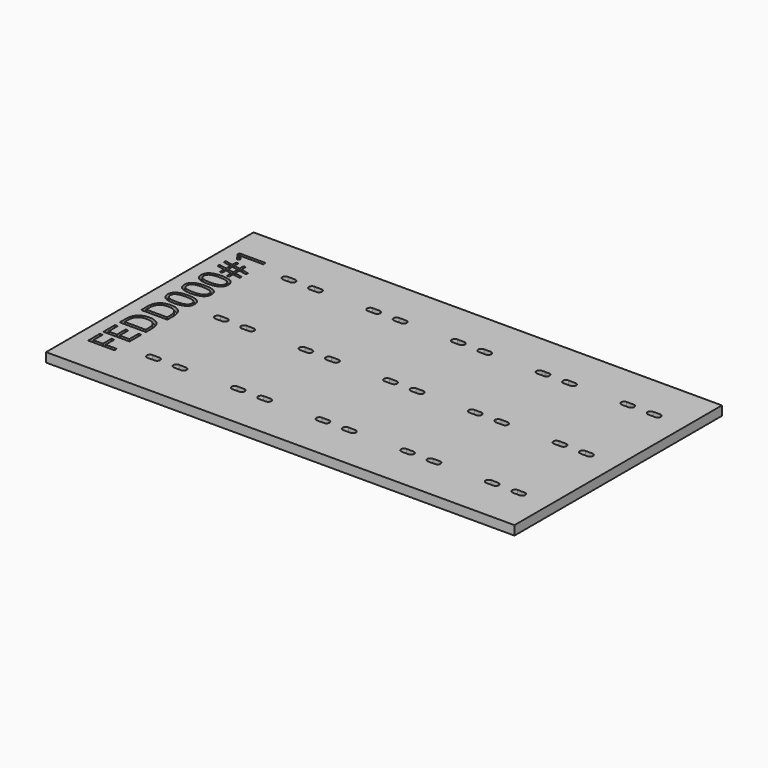
from build123d import *

# Parameters (mm, degrees)
F0_W         = 177
F0_H         = 98
F1_DEPTH     = 3.5
F2_TEXT_SIZE = 13.8888888889
F3_DEPTH     = 1.5
F5_DEPTH     = 3.5
F6_T1_DEPTH  = 3.5


# Not quite as in the source:
# - a fillet or chamfer that OpenCascade refuses, or shapes differently, is made with other operations: its cross-section is extruded or revolved along the edge and cut away or added
# - Text() gives the source's letters only with a copy of the font that has no kerning and outlines rounded to 1/6400 em; it was checked with that copy


with BuildPart() as f1:
    # F0 (on Top) → F1 (new body)
    with BuildSketch(Plane.XY):
        with Locations((0.9526101351, -0.284535466)):
            Rectangle(F0_W, F0_H)
    extrude(amount=F1_DEPTH)

    # F2 (on face) → F3 (cut)
    with BuildSketch(Plane.XY.offset(3.5)):
        with Locations(Location((-72.5473898649, -37.126535466), (0, 0, 90))):
            Text('FEDD000#1', F2_TEXT_SIZE, font='Open Sans', text_align=(TextAlign.LEFT, TextAlign.BOTTOM))
    extrude(amount=-F3_DEPTH, mode=Mode.SUBTRACT)

    # F4 (on face) → F5 (cut, through all)
    with BuildSketch(Plane.XY.offset(3.5)):
        with BuildLine():
            ThreePointArc((-60.5473898649, 30.565464534), (-59.7342170666, 30.9022917356), (-59.3973898649, 31.715464534))
            ThreePointArc((-59.3973898649, 31.715464534), (-59.7342170666, 32.5286373324), (-60.5473898649, 32.865464534))
            ThreePointArc((-60.5473898649, 32.865464534), (-61.6973898649, 31.715464534), (-60.5473898649, 30.565464534))
        make_face()
        with BuildLine():
            ThreePointArc((-60.5473898649, 32.865464534), (-59.7342170666, 32.5286373324), (-59.3973898649, 31.715464534))
            ThreePointArc((-59.3973898649, 31.715464534), (-59.7342170666, 30.9022917356), (-60.5473898649, 30.565464534))
            Line((-60.5473898649, 30.565464534), (-58.0473898649, 30.565464534))
            Line((-58.0473898649, 30.565464534), (-58.0473898649, 32.865464534))
            Line((-58.0473898649, 32.865464534), (-60.5473898649, 32.865464534))
        make_face()
        with BuildLine():
            ThreePointArc((-60.5473898649, 30.565464534), (-61.6973898649, 31.715464534), (-60.5473898649, 32.865464534))
            Line((-60.5473898649, 32.865464534), (-63.0473898649, 32.865464534))
            Line((-63.0473898649, 32.865464534), (-63.0473898649, 30.565464534))
            Line((-63.0473898649, 30.565464534), (-60.5473898649, 30.565464534))
        make_face()
        with BuildLine():
            ThreePointArc((-50.5473898649, 30.565464534), (-49.7342170666, 30.9022917356), (-49.3973898649, 31.715464534))
            ThreePointArc((-49.3973898649, 31.715464534), (-49.7342170666, 32.5286373324), (-50.5473898649, 32.865464534))
            ThreePointArc((-50.5473898649, 32.865464534), (-51.6973898649, 31.715464534), (-50.5473898649, 30.565464534))
        make_face()
        with BuildLine():
            ThreePointArc((-50.5473898649, 32.865464534), (-49.7342170666, 32.5286373324), (-49.3973898649, 31.715464534))
            ThreePointArc((-49.3973898649, 31.715464534), (-49.7342170666, 30.9022917356), (-50.5473898649, 30.565464534))
            Line((-50.5473898649, 30.565464534), (-48.0473898649, 30.565464534))
            Line((-48.0473898649, 30.565464534), (-48.0473898649, 32.865464534))
            Line((-48.0473898649, 32.865464534), (-50.5473898649, 32.865464534))
        make_face()
        with BuildLine():
            ThreePointArc((-50.5473898649, 30.565464534), (-51.6973898649, 31.715464534), (-50.5473898649, 32.865464534))
            Line((-50.5473898649, 32.865464534), (-53.0473898649, 32.865464534))
            Line((-53.0473898649, 32.865464534), (-53.0473898649, 30.565464534))
            Line((-53.0473898649, 30.565464534), (-50.5473898649, 30.565464534))
        make_face()
        with BuildLine():
            ThreePointArc((-28.5473898649, 30.565464534), (-27.7342170666, 30.9022917356), (-27.3973898649, 31.715464534))
            ThreePointArc((-27.3973898649, 31.715464534), (-27.7342170666, 32.5286373324), (-28.5473898649, 32.865464534))
            ThreePointArc((-28.5473898649, 32.865464534), (-29.6973898649, 31.715464534), (-28.5473898649, 30.565464534))
        make_face()
        with BuildLine():
            ThreePointArc((-28.5473898649, 32.865464534), (-27.7342170666, 32.5286373324), (-27.3973898649, 31.715464534))
            ThreePointArc((-27.3973898649, 31.715464534), (-27.7342170666, 30.9022917356), (-28.5473898649, 30.565464534))
            Line((-28.5473898649, 30.565464534), (-26.0473898649, 30.565464534))
            Line((-26.0473898649, 30.565464534), (-26.0473898649, 32.865464534))
            Line((-26.0473898649, 32.865464534), (-28.5473898649, 32.865464534))
        make_face()
        with BuildLine():
            ThreePointArc((-28.5473898649, 30.565464534), (-29.6973898649, 31.715464534), (-28.5473898649, 32.865464534))
            Line((-28.5473898649, 32.865464534), (-31.0473898649, 32.865464534))
            Line((-31.0473898649, 32.865464534), (-31.0473898649, 30.565464534))
            Line((-31.0473898649, 30.565464534), (-28.5473898649, 30.565464534))
        make_face()
        with BuildLine():
            ThreePointArc((-18.5473898649, 30.565464534), (-17.7342170666, 30.9022917356), (-17.3973898649, 31.715464534))
            ThreePointArc((-17.3973898649, 31.715464534), (-17.7342170666, 32.5286373324), (-18.5473898649, 32.865464534))
            ThreePointArc((-18.5473898649, 32.865464534), (-19.6973898649, 31.715464534), (-18.5473898649, 30.565464534))
        make_face()
        with BuildLine():
            ThreePointArc((-18.5473898649, 32.865464534), (-17.7342170666, 32.5286373324), (-17.3973898649, 31.715464534))
            ThreePointArc((-17.3973898649, 31.715464534), (-17.7342170666, 30.9022917356), (-18.5473898649, 30.565464534))
            Line((-18.5473898649, 30.565464534), (-16.0473898649, 30.565464534))
            Line((-16.0473898649, 30.565464534), (-16.0473898649, 32.865464534))
            Line((-16.0473898649, 32.865464534), (-18.5473898649, 32.865464534))
        make_face()
        with BuildLine():
            ThreePointArc((-18.5473898649, 30.565464534), (-19.6973898649, 31.715464534), (-18.5473898649, 32.865464534))
            Line((-18.5473898649, 32.865464534), (-21.0473898649, 32.865464534))
            Line((-21.0473898649, 32.865464534), (-21.0473898649, 30.565464534))
            Line((-21.0473898649, 30.565464534), (-18.5473898649, 30.565464534))
        make_face()
        with BuildLine():
            ThreePointArc((3.4526101351, 30.565464534), (4.2657829334, 30.9022917356), (4.6026101351, 31.715464534))
            ThreePointArc((4.6026101351, 31.715464534), (4.2657829334, 32.5286373324), (3.4526101351, 32.865464534))
            ThreePointArc((3.4526101351, 32.865464534), (2.3026101351, 31.715464534), (3.4526101351, 30.565464534))
        make_face()
        with BuildLine():
            ThreePointArc((3.4526101351, 32.865464534), (4.2657829334, 32.5286373324), (4.6026101351, 31.715464534))
            ThreePointArc((4.6026101351, 31.715464534), (4.2657829334, 30.9022917356), (3.4526101351, 30.565464534))
            Line((3.4526101351, 30.565464534), (5.9526101351, 30.565464534))
            Line((5.9526101351, 30.565464534), (5.9526101351, 32.865464534))
            Line((5.9526101351, 32.865464534), (3.4526101351, 32.865464534))
        make_face()
        with BuildLine():
            ThreePointArc((3.4526101351, 30.565464534), (2.3026101351, 31.715464534), (3.4526101351, 32.865464534))
            Line((3.4526101351, 32.865464534), (0.9526101351, 32.865464534))
            Line((0.9526101351, 32.865464534), (0.9526101351, 30.565464534))
            Line((0.9526101351, 30.565464534), (3.4526101351, 30.565464534))
        make_face()
        with BuildLine():
            ThreePointArc((13.4526101351, 30.565464534), (14.2657829334, 30.9022917356), (14.6026101351, 31.715464534))
            ThreePointArc((14.6026101351, 31.715464534), (14.2657829334, 32.5286373324), (13.4526101351, 32.865464534))
            ThreePointArc((13.4526101351, 32.865464534), (12.3026101351, 31.715464534), (13.4526101351, 30.565464534))
        make_face()
        with BuildLine():
            ThreePointArc((13.4526101351, 32.865464534), (14.2657829334, 32.5286373324), (14.6026101351, 31.715464534))
            ThreePointArc((14.6026101351, 31.715464534), (14.2657829334, 30.9022917356), (13.4526101351, 30.565464534))
            Line((13.4526101351, 30.565464534), (15.9526101351, 30.565464534))
            Line((15.9526101351, 30.565464534), (15.9526101351, 32.865464534))
            Line((15.9526101351, 32.865464534), (13.4526101351, 32.865464534))
        make_face()
        with BuildLine():
            ThreePointArc((13.4526101351, 30.565464534), (12.3026101351, 31.715464534), (13.4526101351, 32.865464534))
            Line((13.4526101351, 32.865464534), (10.9526101351, 32.865464534))
            Line((10.9526101351, 32.865464534), (10.9526101351, 30.565464534))
            Line((10.9526101351, 30.565464534), (13.4526101351, 30.565464534))
        make_face()
        with BuildLine():
            ThreePointArc((35.23906857, 32.845464534), (34.7188093446, 30.8300062346), (36.6026101351, 31.715464534))
            ThreePointArc((36.6026101351, 31.715464534), (36.3380684344, 32.4492653245), (35.6661517001, 32.845464534))
            Line((35.6661517001, 32.845464534), (35.23906857, 32.845464534))
        make_face()
        with BuildLine():
            ThreePointArc((35.6661517001, 32.845464534), (36.3380684344, 32.4492653245), (36.6026101351, 31.715464534))
            ThreePointArc((36.6026101351, 31.715464534), (34.7188093446, 30.8300062346), (35.23906857, 32.845464534))
            Line((35.23906857, 32.845464534), (32.9526101351, 32.845464534))
            Line((32.9526101351, 32.845464534), (32.9526101351, 30.545464534))
            Line((32.9526101351, 30.545464534), (37.9526101351, 30.545464534))
            Line((37.9526101351, 30.545464534), (37.9526101351, 32.845464534))
            Line((37.9526101351, 32.845464534), (35.6661517001, 32.845464534))
        make_face()
        with BuildLine():
            Line((35.23906857, 32.845464534), (35.6661517001, 32.845464534))
            ThreePointArc((35.6661517001, 32.845464534), (35.4526101351, 32.865464534), (35.23906857, 32.845464534))
        make_face()
        with BuildLine():
            ThreePointArc((45.4526101351, 30.565464534), (46.2657829334, 30.9022917356), (46.6026101351, 31.715464534))
            ThreePointArc((46.6026101351, 31.715464534), (46.2657829334, 32.5286373324), (45.4526101351, 32.865464534))
            ThreePointArc((45.4526101351, 32.865464534), (44.3026101351, 31.715464534), (45.4526101351, 30.565464534))
        make_face()
        with BuildLine():
            ThreePointArc((45.4526101351, 32.865464534), (46.2657829334, 32.5286373324), (46.6026101351, 31.715464534))
            ThreePointArc((46.6026101351, 31.715464534), (46.2657829334, 30.9022917356), (45.4526101351, 30.565464534))
            Line((45.4526101351, 30.565464534), (47.9526101351, 30.565464534))
            Line((47.9526101351, 30.565464534), (47.9526101351, 32.865464534))
            Line((47.9526101351, 32.865464534), (45.4526101351, 32.865464534))
        make_face()
        with BuildLine():
            ThreePointArc((45.4526101351, 30.565464534), (44.3026101351, 31.715464534), (45.4526101351, 32.865464534))
            Line((45.4526101351, 32.865464534), (42.9526101351, 32.865464534))
            Line((42.9526101351, 32.865464534), (42.9526101351, 30.565464534))
            Line((42.9526101351, 30.565464534), (45.4526101351, 30.565464534))
        make_face()
        with BuildLine():
            ThreePointArc((67.4526101351, 30.565464534), (68.2657829334, 30.9022917356), (68.6026101351, 31.715464534))
            ThreePointArc((68.6026101351, 31.715464534), (68.2657829334, 32.5286373324), (67.4526101351, 32.865464534))
            ThreePointArc((67.4526101351, 32.865464534), (66.3026101351, 31.715464534), (67.4526101351, 30.565464534))
        make_face()
        with BuildLine():
            ThreePointArc((67.4526101351, 32.865464534), (68.2657829334, 32.5286373324), (68.6026101351, 31.715464534))
            ThreePointArc((68.6026101351, 31.715464534), (68.2657829334, 30.9022917356), (67.4526101351, 30.565464534))
            Line((67.4526101351, 30.565464534), (69.9526101351, 30.565464534))
            Line((69.9526101351, 30.565464534), (69.9526101351, 32.865464534))
            Line((69.9526101351, 32.865464534), (67.4526101351, 32.865464534))
        make_face()
        with BuildLine():
            ThreePointArc((67.4526101351, 30.565464534), (66.3026101351, 31.715464534), (67.4526101351, 32.865464534))
            Line((67.4526101351, 32.865464534), (64.9526101351, 32.865464534))
            Line((64.9526101351, 32.865464534), (64.9526101351, 30.565464534))
            Line((64.9526101351, 30.565464534), (67.4526101351, 30.565464534))
        make_face()
        with BuildLine():
            ThreePointArc((77.4526101351, 30.565464534), (78.2657829334, 30.9022917356), (78.6026101351, 31.715464534))
            ThreePointArc((78.6026101351, 31.715464534), (78.2657829334, 32.5286373324), (77.4526101351, 32.865464534))
            ThreePointArc((77.4526101351, 32.865464534), (76.3026101351, 31.715464534), (77.4526101351, 30.565464534))
        make_face()
        with BuildLine():
            ThreePointArc((77.4526101351, 32.865464534), (78.2657829334, 32.5286373324), (78.6026101351, 31.715464534))
            ThreePointArc((78.6026101351, 31.715464534), (78.2657829334, 30.9022917356), (77.4526101351, 30.565464534))
            Line((77.4526101351, 30.565464534), (79.9526101351, 30.565464534))
            Line((79.9526101351, 30.565464534), (79.9526101351, 32.865464534))
            Line((79.9526101351, 32.865464534), (77.4526101351, 32.865464534))
        make_face()
        with BuildLine():
            ThreePointArc((77.4526101351, 30.565464534), (76.3026101351, 31.715464534), (77.4526101351, 32.865464534))
            Line((77.4526101351, 32.865464534), (74.9526101351, 32.865464534))
            Line((74.9526101351, 32.865464534), (74.9526101351, 30.565464534))
            Line((74.9526101351, 30.565464534), (77.4526101351, 30.565464534))
        make_face()
        with BuildLine():
            ThreePointArc((-60.5473898649, -1.434535466), (-59.7342170666, -1.0977082644), (-59.3973898649, -0.284535466))
            ThreePointArc((-59.3973898649, -0.284535466), (-59.7342170666, 0.5286373324), (-60.5473898649, 0.865464534))
            ThreePointArc((-60.5473898649, 0.865464534), (-61.6973898649, -0.284535466), (-60.5473898649, -1.434535466))
        make_face()
        with BuildLine():
            ThreePointArc((-60.5473898649, 0.865464534), (-59.7342170666, 0.5286373324), (-59.3973898649, -0.284535466))
            ThreePointArc((-59.3973898649, -0.284535466), (-59.7342170666, -1.0977082644), (-60.5473898649, -1.434535466))
            Line((-60.5473898649, -1.434535466), (-58.0473898649, -1.434535466))
            Line((-58.0473898649, -1.434535466), (-58.0473898649, 0.865464534))
            Line((-58.0473898649, 0.865464534), (-60.5473898649, 0.865464534))
        make_face()
        with BuildLine():
            ThreePointArc((-60.5473898649, -1.434535466), (-61.6973898649, -0.284535466), (-60.5473898649, 0.865464534))
            Line((-60.5473898649, 0.865464534), (-63.0473898649, 0.865464534))
            Line((-63.0473898649, 0.865464534), (-63.0473898649, -1.434535466))
            Line((-63.0473898649, -1.434535466), (-60.5473898649, -1.434535466))
        make_face()
        with BuildLine():
            ThreePointArc((-50.5473898649, -1.434535466), (-49.7342170666, -1.0977082644), (-49.3973898649, -0.284535466))
            ThreePointArc((-49.3973898649, -0.284535466), (-49.7342170666, 0.5286373324), (-50.5473898649, 0.865464534))
            ThreePointArc((-50.5473898649, 0.865464534), (-51.6973898649, -0.284535466), (-50.5473898649, -1.434535466))
        make_face()
        with BuildLine():
            ThreePointArc((-50.5473898649, 0.865464534), (-49.7342170666, 0.5286373324), (-49.3973898649, -0.284535466))
            ThreePointArc((-49.3973898649, -0.284535466), (-49.7342170666, -1.0977082644), (-50.5473898649, -1.434535466))
            Line((-50.5473898649, -1.434535466), (-48.0473898649, -1.434535466))
            Line((-48.0473898649, -1.434535466), (-48.0473898649, 0.865464534))
            Line((-48.0473898649, 0.865464534), (-50.5473898649, 0.865464534))
        make_face()
        with BuildLine():
            ThreePointArc((-50.5473898649, -1.434535466), (-51.6973898649, -0.284535466), (-50.5473898649, 0.865464534))
            Line((-50.5473898649, 0.865464534), (-53.0473898649, 0.865464534))
            Line((-53.0473898649, 0.865464534), (-53.0473898649, -1.434535466))
            Line((-53.0473898649, -1.434535466), (-50.5473898649, -1.434535466))
        make_face()
        with BuildLine():
            ThreePointArc((-28.5473898649, -1.434535466), (-27.7342170666, -1.0977082644), (-27.3973898649, -0.284535466))
            ThreePointArc((-27.3973898649, -0.284535466), (-27.7342170666, 0.5286373324), (-28.5473898649, 0.865464534))
            ThreePointArc((-28.5473898649, 0.865464534), (-29.6973898649, -0.284535466), (-28.5473898649, -1.434535466))
        make_face()
        with BuildLine():
            ThreePointArc((-28.5473898649, 0.865464534), (-27.7342170666, 0.5286373324), (-27.3973898649, -0.284535466))
            ThreePointArc((-27.3973898649, -0.284535466), (-27.7342170666, -1.0977082644), (-28.5473898649, -1.434535466))
            Line((-28.5473898649, -1.434535466), (-26.0473898649, -1.434535466))
            Line((-26.0473898649, -1.434535466), (-26.0473898649, 0.865464534))
            Line((-26.0473898649, 0.865464534), (-28.5473898649, 0.865464534))
        make_face()
        with BuildLine():
            ThreePointArc((-28.5473898649, -1.434535466), (-29.6973898649, -0.284535466), (-28.5473898649, 0.865464534))
            Line((-28.5473898649, 0.865464534), (-31.0473898649, 0.865464534))
            Line((-31.0473898649, 0.865464534), (-31.0473898649, -1.434535466))
            Line((-31.0473898649, -1.434535466), (-28.5473898649, -1.434535466))
        make_face()
        with BuildLine():
            ThreePointArc((-18.5473898649, -1.434535466), (-17.7342170666, -1.0977082644), (-17.3973898649, -0.284535466))
            ThreePointArc((-17.3973898649, -0.284535466), (-17.7342170666, 0.5286373324), (-18.5473898649, 0.865464534))
            ThreePointArc((-18.5473898649, 0.865464534), (-19.6973898649, -0.284535466), (-18.5473898649, -1.434535466))
        make_face()
        with BuildLine():
            ThreePointArc((-18.5473898649, 0.865464534), (-17.7342170666, 0.5286373324), (-17.3973898649, -0.284535466))
            ThreePointArc((-17.3973898649, -0.284535466), (-17.7342170666, -1.0977082644), (-18.5473898649, -1.434535466))
            Line((-18.5473898649, -1.434535466), (-16.0473898649, -1.434535466))
            Line((-16.0473898649, -1.434535466), (-16.0473898649, 0.865464534))
            Line((-16.0473898649, 0.865464534), (-18.5473898649, 0.865464534))
        make_face()
        with BuildLine():
            ThreePointArc((-18.5473898649, -1.434535466), (-19.6973898649, -0.284535466), (-18.5473898649, 0.865464534))
            Line((-18.5473898649, 0.865464534), (-21.0473898649, 0.865464534))
            Line((-21.0473898649, 0.865464534), (-21.0473898649, -1.434535466))
            Line((-21.0473898649, -1.434535466), (-18.5473898649, -1.434535466))
        make_face()
        with BuildLine():
            ThreePointArc((3.4526101351, -1.434535466), (4.2657829334, -1.0977082644), (4.6026101351, -0.284535466))
            ThreePointArc((4.6026101351, -0.284535466), (4.2657829334, 0.5286373324), (3.4526101351, 0.865464534))
            ThreePointArc((3.4526101351, 0.865464534), (2.3026101351, -0.284535466), (3.4526101351, -1.434535466))
        make_face()
        with BuildLine():
            ThreePointArc((3.4526101351, 0.865464534), (4.2657829334, 0.5286373324), (4.6026101351, -0.284535466))
            ThreePointArc((4.6026101351, -0.284535466), (4.2657829334, -1.0977082644), (3.4526101351, -1.434535466))
            Line((3.4526101351, -1.434535466), (5.9526101351, -1.434535466))
            Line((5.9526101351, -1.434535466), (5.9526101351, 0.865464534))
            Line((5.9526101351, 0.865464534), (3.4526101351, 0.865464534))
        make_face()
        with BuildLine():
            ThreePointArc((3.4526101351, -1.434535466), (2.3026101351, -0.284535466), (3.4526101351, 0.865464534))
            Line((3.4526101351, 0.865464534), (0.9526101351, 0.865464534))
            Line((0.9526101351, 0.865464534), (0.9526101351, -1.434535466))
            Line((0.9526101351, -1.434535466), (3.4526101351, -1.434535466))
        make_face()
        with BuildLine():
            ThreePointArc((13.4526101351, -1.434535466), (14.2657829334, -1.0977082644), (14.6026101351, -0.284535466))
            ThreePointArc((14.6026101351, -0.284535466), (14.2657829334, 0.5286373324), (13.4526101351, 0.865464534))
            ThreePointArc((13.4526101351, 0.865464534), (12.3026101351, -0.284535466), (13.4526101351, -1.434535466))
        make_face()
        with BuildLine():
            ThreePointArc((13.4526101351, 0.865464534), (14.2657829334, 0.5286373324), (14.6026101351, -0.284535466))
            ThreePointArc((14.6026101351, -0.284535466), (14.2657829334, -1.0977082644), (13.4526101351, -1.434535466))
            Line((13.4526101351, -1.434535466), (15.9526101351, -1.434535466))
            Line((15.9526101351, -1.434535466), (15.9526101351, 0.865464534))
            Line((15.9526101351, 0.865464534), (13.4526101351, 0.865464534))
        make_face()
        with BuildLine():
            ThreePointArc((13.4526101351, -1.434535466), (12.3026101351, -0.284535466), (13.4526101351, 0.865464534))
            Line((13.4526101351, 0.865464534), (10.9526101351, 0.865464534))
            Line((10.9526101351, 0.865464534), (10.9526101351, -1.434535466))
            Line((10.9526101351, -1.434535466), (13.4526101351, -1.434535466))
        make_face()
        with BuildLine():
            ThreePointArc((35.4526101351, -1.434535466), (36.2657829334, -1.0977082644), (36.6026101351, -0.284535466))
            ThreePointArc((36.6026101351, -0.284535466), (36.2657829334, 0.5286373324), (35.4526101351, 0.865464534))
            ThreePointArc((35.4526101351, 0.865464534), (34.3026101351, -0.284535466), (35.4526101351, -1.434535466))
        make_face()
        with BuildLine():
            ThreePointArc((35.4526101351, 0.865464534), (36.2657829334, 0.5286373324), (36.6026101351, -0.284535466))
            ThreePointArc((36.6026101351, -0.284535466), (36.2657829334, -1.0977082644), (35.4526101351, -1.434535466))
            Line((35.4526101351, -1.434535466), (37.9526101351, -1.434535466))
            Line((37.9526101351, -1.434535466), (37.9526101351, 0.865464534))
            Line((37.9526101351, 0.865464534), (35.4526101351, 0.865464534))
        make_face()
        with BuildLine():
            ThreePointArc((35.4526101351, -1.434535466), (34.3026101351, -0.284535466), (35.4526101351, 0.865464534))
            Line((35.4526101351, 0.865464534), (32.9526101351, 0.865464534))
            Line((32.9526101351, 0.865464534), (32.9526101351, -1.434535466))
            Line((32.9526101351, -1.434535466), (35.4526101351, -1.434535466))
        make_face()
        with BuildLine():
            ThreePointArc((45.4526101351, -1.434535466), (46.2657829334, -1.0977082644), (46.6026101351, -0.284535466))
            ThreePointArc((46.6026101351, -0.284535466), (46.2657829334, 0.5286373324), (45.4526101351, 0.865464534))
            ThreePointArc((45.4526101351, 0.865464534), (44.3026101351, -0.284535466), (45.4526101351, -1.434535466))
        make_face()
        with BuildLine():
            ThreePointArc((45.4526101351, 0.865464534), (46.2657829334, 0.5286373324), (46.6026101351, -0.284535466))
            ThreePointArc((46.6026101351, -0.284535466), (46.2657829334, -1.0977082644), (45.4526101351, -1.434535466))
            Line((45.4526101351, -1.434535466), (47.9526101351, -1.434535466))
            Line((47.9526101351, -1.434535466), (47.9526101351, 0.865464534))
            Line((47.9526101351, 0.865464534), (45.4526101351, 0.865464534))
        make_face()
        with BuildLine():
            ThreePointArc((45.4526101351, -1.434535466), (44.3026101351, -0.284535466), (45.4526101351, 0.865464534))
            Line((45.4526101351, 0.865464534), (42.9526101351, 0.865464534))
            Line((42.9526101351, 0.865464534), (42.9526101351, -1.434535466))
            Line((42.9526101351, -1.434535466), (45.4526101351, -1.434535466))
        make_face()
        with BuildLine():
            ThreePointArc((67.4526101351, -1.434535466), (68.2657829334, -1.0977082644), (68.6026101351, -0.284535466))
            ThreePointArc((68.6026101351, -0.284535466), (68.2657829334, 0.5286373324), (67.4526101351, 0.865464534))
            ThreePointArc((67.4526101351, 0.865464534), (66.3026101351, -0.284535466), (67.4526101351, -1.434535466))
        make_face()
        with BuildLine():
            ThreePointArc((67.4526101351, 0.865464534), (68.2657829334, 0.5286373324), (68.6026101351, -0.284535466))
            ThreePointArc((68.6026101351, -0.284535466), (68.2657829334, -1.0977082644), (67.4526101351, -1.434535466))
            Line((67.4526101351, -1.434535466), (69.9526101351, -1.434535466))
            Line((69.9526101351, -1.434535466), (69.9526101351, 0.865464534))
            Line((69.9526101351, 0.865464534), (67.4526101351, 0.865464534))
        make_face()
        with BuildLine():
            ThreePointArc((67.4526101351, -1.434535466), (66.3026101351, -0.284535466), (67.4526101351, 0.865464534))
            Line((67.4526101351, 0.865464534), (64.9526101351, 0.865464534))
            Line((64.9526101351, 0.865464534), (64.9526101351, -1.434535466))
            Line((64.9526101351, -1.434535466), (67.4526101351, -1.434535466))
        make_face()
        with BuildLine():
            ThreePointArc((77.4526101351, -1.434535466), (78.2657829334, -1.0977082644), (78.6026101351, -0.284535466))
            ThreePointArc((78.6026101351, -0.284535466), (78.2657829334, 0.5286373324), (77.4526101351, 0.865464534))
            ThreePointArc((77.4526101351, 0.865464534), (76.3026101351, -0.284535466), (77.4526101351, -1.434535466))
        make_face()
        with BuildLine():
            ThreePointArc((77.4526101351, 0.865464534), (78.2657829334, 0.5286373324), (78.6026101351, -0.284535466))
            ThreePointArc((78.6026101351, -0.284535466), (78.2657829334, -1.0977082644), (77.4526101351, -1.434535466))
            Line((77.4526101351, -1.434535466), (79.9526101351, -1.434535466))
            Line((79.9526101351, -1.434535466), (79.9526101351, 0.865464534))
            Line((79.9526101351, 0.865464534), (77.4526101351, 0.865464534))
        make_face()
        with BuildLine():
            ThreePointArc((77.4526101351, -1.434535466), (76.3026101351, -0.284535466), (77.4526101351, 0.865464534))
            Line((77.4526101351, 0.865464534), (74.9526101351, 0.865464534))
            Line((74.9526101351, 0.865464534), (74.9526101351, -1.434535466))
            Line((74.9526101351, -1.434535466), (77.4526101351, -1.434535466))
        make_face()
        with BuildLine():
            ThreePointArc((-60.5473898649, -33.434535466), (-59.7342170666, -33.0977082644), (-59.3973898649, -32.284535466))
            ThreePointArc((-59.3973898649, -32.284535466), (-59.7342170666, -31.4713626676), (-60.5473898649, -31.134535466))
            ThreePointArc((-60.5473898649, -31.134535466), (-61.6973898649, -32.284535466), (-60.5473898649, -33.434535466))
        make_face()
        with BuildLine():
            ThreePointArc((-60.5473898649, -31.134535466), (-59.7342170666, -31.4713626676), (-59.3973898649, -32.284535466))
            ThreePointArc((-59.3973898649, -32.284535466), (-59.7342170666, -33.0977082644), (-60.5473898649, -33.434535466))
            Line((-60.5473898649, -33.434535466), (-58.0473898649, -33.434535466))
            Line((-58.0473898649, -33.434535466), (-58.0473898649, -31.134535466))
            Line((-58.0473898649, -31.134535466), (-60.5473898649, -31.134535466))
        make_face()
        with BuildLine():
            ThreePointArc((-60.5473898649, -33.434535466), (-61.6973898649, -32.284535466), (-60.5473898649, -31.134535466))
            Line((-60.5473898649, -31.134535466), (-63.0473898649, -31.134535466))
            Line((-63.0473898649, -31.134535466), (-63.0473898649, -33.434535466))
            Line((-63.0473898649, -33.434535466), (-60.5473898649, -33.434535466))
        make_face()
        with BuildLine():
            ThreePointArc((-50.5473898649, -33.434535466), (-49.7342170666, -33.0977082644), (-49.3973898649, -32.284535466))
            ThreePointArc((-49.3973898649, -32.284535466), (-49.7342170666, -31.4713626676), (-50.5473898649, -31.134535466))
            ThreePointArc((-50.5473898649, -31.134535466), (-51.6973898649, -32.284535466), (-50.5473898649, -33.434535466))
        make_face()
        with BuildLine():
            ThreePointArc((-50.5473898649, -31.134535466), (-49.7342170666, -31.4713626676), (-49.3973898649, -32.284535466))
            ThreePointArc((-49.3973898649, -32.284535466), (-49.7342170666, -33.0977082644), (-50.5473898649, -33.434535466))
            Line((-50.5473898649, -33.434535466), (-48.0473898649, -33.434535466))
            Line((-48.0473898649, -33.434535466), (-48.0473898649, -31.134535466))
            Line((-48.0473898649, -31.134535466), (-50.5473898649, -31.134535466))
        make_face()
        with BuildLine():
            ThreePointArc((-50.5473898649, -33.434535466), (-51.6973898649, -32.284535466), (-50.5473898649, -31.134535466))
            Line((-50.5473898649, -31.134535466), (-53.0473898649, -31.134535466))
            Line((-53.0473898649, -31.134535466), (-53.0473898649, -33.434535466))
            Line((-53.0473898649, -33.434535466), (-50.5473898649, -33.434535466))
        make_face()
        with BuildLine():
            ThreePointArc((-28.5473898649, -33.434535466), (-27.7342170666, -33.0977082644), (-27.3973898649, -32.284535466))
            ThreePointArc((-27.3973898649, -32.284535466), (-27.7342170666, -31.4713626676), (-28.5473898649, -31.134535466))
            ThreePointArc((-28.5473898649, -31.134535466), (-29.6973898649, -32.284535466), (-28.5473898649, -33.434535466))
        make_face()
        with BuildLine():
            ThreePointArc((-28.5473898649, -31.134535466), (-27.7342170666, -31.4713626676), (-27.3973898649, -32.284535466))
            ThreePointArc((-27.3973898649, -32.284535466), (-27.7342170666, -33.0977082644), (-28.5473898649, -33.434535466))
            Line((-28.5473898649, -33.434535466), (-26.0473898649, -33.434535466))
            Line((-26.0473898649, -33.434535466), (-26.0473898649, -31.134535466))
            Line((-26.0473898649, -31.134535466), (-28.5473898649, -31.134535466))
        make_face()
        with BuildLine():
            ThreePointArc((-28.5473898649, -33.434535466), (-29.6973898649, -32.284535466), (-28.5473898649, -31.134535466))
            Line((-28.5473898649, -31.134535466), (-31.0473898649, -31.134535466))
            Line((-31.0473898649, -31.134535466), (-31.0473898649, -33.434535466))
            Line((-31.0473898649, -33.434535466), (-28.5473898649, -33.434535466))
        make_face()
        with BuildLine():
            ThreePointArc((-18.5473898649, -33.434535466), (-17.7342170666, -33.0977082644), (-17.3973898649, -32.284535466))
            ThreePointArc((-17.3973898649, -32.284535466), (-17.7342170666, -31.4713626676), (-18.5473898649, -31.134535466))
            ThreePointArc((-18.5473898649, -31.134535466), (-19.6973898649, -32.284535466), (-18.5473898649, -33.434535466))
        make_face()
        with BuildLine():
            ThreePointArc((-18.5473898649, -31.134535466), (-17.7342170666, -31.4713626676), (-17.3973898649, -32.284535466))
            ThreePointArc((-17.3973898649, -32.284535466), (-17.7342170666, -33.0977082644), (-18.5473898649, -33.434535466))
            Line((-18.5473898649, -33.434535466), (-16.0473898649, -33.434535466))
            Line((-16.0473898649, -33.434535466), (-16.0473898649, -31.134535466))
            Line((-16.0473898649, -31.134535466), (-18.5473898649, -31.134535466))
        make_face()
        with BuildLine():
            ThreePointArc((-18.5473898649, -33.434535466), (-19.6973898649, -32.284535466), (-18.5473898649, -31.134535466))
            Line((-18.5473898649, -31.134535466), (-21.0473898649, -31.134535466))
            Line((-21.0473898649, -31.134535466), (-21.0473898649, -33.434535466))
            Line((-21.0473898649, -33.434535466), (-18.5473898649, -33.434535466))
        make_face()
        with BuildLine():
            ThreePointArc((3.4526101351, -33.434535466), (4.2657829334, -33.0977082644), (4.6026101351, -32.284535466))
            ThreePointArc((4.6026101351, -32.284535466), (4.2657829334, -31.4713626676), (3.4526101351, -31.134535466))
            ThreePointArc((3.4526101351, -31.134535466), (2.3026101351, -32.284535466), (3.4526101351, -33.434535466))
        make_face()
        with BuildLine():
            ThreePointArc((3.4526101351, -31.134535466), (4.2657829334, -31.4713626676), (4.6026101351, -32.284535466))
            ThreePointArc((4.6026101351, -32.284535466), (4.2657829334, -33.0977082644), (3.4526101351, -33.434535466))
            Line((3.4526101351, -33.434535466), (5.9526101351, -33.434535466))
            Line((5.9526101351, -33.434535466), (5.9526101351, -31.134535466))
            Line((5.9526101351, -31.134535466), (3.4526101351, -31.134535466))
        make_face()
        with BuildLine():
            ThreePointArc((3.4526101351, -33.434535466), (2.3026101351, -32.284535466), (3.4526101351, -31.134535466))
            Line((3.4526101351, -31.134535466), (0.9526101351, -31.134535466))
            Line((0.9526101351, -31.134535466), (0.9526101351, -33.434535466))
            Line((0.9526101351, -33.434535466), (3.4526101351, -33.434535466))
        make_face()
        with BuildLine():
            ThreePointArc((13.4526101351, -33.434535466), (14.2657829334, -33.0977082644), (14.6026101351, -32.284535466))
            ThreePointArc((14.6026101351, -32.284535466), (14.2657829334, -31.4713626676), (13.4526101351, -31.134535466))
            ThreePointArc((13.4526101351, -31.134535466), (12.3026101351, -32.284535466), (13.4526101351, -33.434535466))
        make_face()
        with BuildLine():
            ThreePointArc((13.4526101351, -31.134535466), (14.2657829334, -31.4713626676), (14.6026101351, -32.284535466))
            ThreePointArc((14.6026101351, -32.284535466), (14.2657829334, -33.0977082644), (13.4526101351, -33.434535466))
            Line((13.4526101351, -33.434535466), (15.9526101351, -33.434535466))
            Line((15.9526101351, -33.434535466), (15.9526101351, -31.134535466))
            Line((15.9526101351, -31.134535466), (13.4526101351, -31.134535466))
        make_face()
        with BuildLine():
            ThreePointArc((13.4526101351, -33.434535466), (12.3026101351, -32.284535466), (13.4526101351, -31.134535466))
            Line((13.4526101351, -31.134535466), (10.9526101351, -31.134535466))
            Line((10.9526101351, -31.134535466), (10.9526101351, -33.434535466))
            Line((10.9526101351, -33.434535466), (13.4526101351, -33.434535466))
        make_face()
        with BuildLine():
            ThreePointArc((35.4526101351, -33.434535466), (36.2657829334, -33.0977082644), (36.6026101351, -32.284535466))
            ThreePointArc((36.6026101351, -32.284535466), (36.2657829334, -31.4713626676), (35.4526101351, -31.134535466))
            ThreePointArc((35.4526101351, -31.134535466), (34.3026101351, -32.284535466), (35.4526101351, -33.434535466))
        make_face()
        with BuildLine():
            ThreePointArc((35.4526101351, -31.134535466), (36.2657829334, -31.4713626676), (36.6026101351, -32.284535466))
            ThreePointArc((36.6026101351, -32.284535466), (36.2657829334, -33.0977082644), (35.4526101351, -33.434535466))
            Line((35.4526101351, -33.434535466), (37.9526101351, -33.434535466))
            Line((37.9526101351, -33.434535466), (37.9526101351, -31.134535466))
            Line((37.9526101351, -31.134535466), (35.4526101351, -31.134535466))
        make_face()
        with BuildLine():
            ThreePointArc((35.4526101351, -33.434535466), (34.3026101351, -32.284535466), (35.4526101351, -31.134535466))
            Line((35.4526101351, -31.134535466), (32.9526101351, -31.134535466))
            Line((32.9526101351, -31.134535466), (32.9526101351, -33.434535466))
            Line((32.9526101351, -33.434535466), (35.4526101351, -33.434535466))
        make_face()
        with BuildLine():
            ThreePointArc((45.4526101351, -33.434535466), (46.2657829334, -33.0977082644), (46.6026101351, -32.284535466))
            ThreePointArc((46.6026101351, -32.284535466), (46.2657829334, -31.4713626676), (45.4526101351, -31.134535466))
            ThreePointArc((45.4526101351, -31.134535466), (44.3026101351, -32.284535466), (45.4526101351, -33.434535466))
        make_face()
        with BuildLine():
            ThreePointArc((45.4526101351, -31.134535466), (46.2657829334, -31.4713626676), (46.6026101351, -32.284535466))
            ThreePointArc((46.6026101351, -32.284535466), (46.2657829334, -33.0977082644), (45.4526101351, -33.434535466))
            Line((45.4526101351, -33.434535466), (47.9526101351, -33.434535466))
            Line((47.9526101351, -33.434535466), (47.9526101351, -31.134535466))
            Line((47.9526101351, -31.134535466), (45.4526101351, -31.134535466))
        make_face()
        with BuildLine():
            ThreePointArc((45.4526101351, -33.434535466), (44.3026101351, -32.284535466), (45.4526101351, -31.134535466))
            Line((45.4526101351, -31.134535466), (42.9526101351, -31.134535466))
            Line((42.9526101351, -31.134535466), (42.9526101351, -33.434535466))
            Line((42.9526101351, -33.434535466), (45.4526101351, -33.434535466))
        make_face()
        with BuildLine():
            ThreePointArc((67.4526101351, -33.434535466), (68.2657829334, -33.0977082644), (68.6026101351, -32.284535466))
            ThreePointArc((68.6026101351, -32.284535466), (68.2657829334, -31.4713626676), (67.4526101351, -31.134535466))
            ThreePointArc((67.4526101351, -31.134535466), (66.3026101351, -32.284535466), (67.4526101351, -33.434535466))
        make_face()
        with BuildLine():
            ThreePointArc((67.4526101351, -31.134535466), (68.2657829334, -31.4713626676), (68.6026101351, -32.284535466))
            ThreePointArc((68.6026101351, -32.284535466), (68.2657829334, -33.0977082644), (67.4526101351, -33.434535466))
            Line((67.4526101351, -33.434535466), (69.9526101351, -33.434535466))
            Line((69.9526101351, -33.434535466), (69.9526101351, -31.134535466))
            Line((69.9526101351, -31.134535466), (67.4526101351, -31.134535466))
        make_face()
        with BuildLine():
            ThreePointArc((67.4526101351, -33.434535466), (66.3026101351, -32.284535466), (67.4526101351, -31.134535466))
            Line((67.4526101351, -31.134535466), (64.9526101351, -31.134535466))
            Line((64.9526101351, -31.134535466), (64.9526101351, -33.434535466))
            Line((64.9526101351, -33.434535466), (67.4526101351, -33.434535466))
        make_face()
        with BuildLine():
            ThreePointArc((77.4526101351, -33.434535466), (78.2657829334, -33.0977082644), (78.6026101351, -32.284535466))
            ThreePointArc((78.6026101351, -32.284535466), (78.2657829334, -31.4713626676), (77.4526101351, -31.134535466))
            ThreePointArc((77.4526101351, -31.134535466), (76.3026101351, -32.284535466), (77.4526101351, -33.434535466))
        make_face()
        with BuildLine():
            ThreePointArc((77.4526101351, -31.134535466), (78.2657829334, -31.4713626676), (78.6026101351, -32.284535466))
            ThreePointArc((78.6026101351, -32.284535466), (78.2657829334, -33.0977082644), (77.4526101351, -33.434535466))
            Line((77.4526101351, -33.434535466), (79.9526101351, -33.434535466))
            Line((79.9526101351, -33.434535466), (79.9526101351, -31.134535466))
            Line((79.9526101351, -31.134535466), (77.4526101351, -31.134535466))
        make_face()
        with BuildLine():
            ThreePointArc((77.4526101351, -33.434535466), (76.3026101351, -32.284535466), (77.4526101351, -31.134535466))
            Line((77.4526101351, -31.134535466), (74.9526101351, -31.134535466))
            Line((74.9526101351, -31.134535466), (74.9526101351, -33.434535466))
            Line((74.9526101351, -33.434535466), (77.4526101351, -33.434535466))
        make_face()
    extrude(amount=-F5_DEPTH, mode=Mode.SUBTRACT)

    # F6: fillet of radius 1.2 on 120 edges, made by hand

    # F6_s2 → F6_t1 (join)
    with BuildSketch(Plane.XY):
        with BuildLine():
            ThreePointArc((-51.8473898649, 32.865464534), (-52.6959180023, 32.5139926714), (-53.0473898649, 31.665464534))
            Line((-53.0473898649, 31.665464534), (-53.0473898649, 32.865464534))
            Line((-53.0473898649, 32.865464534), (-51.8473898649, 32.865464534))
        make_face()
        with BuildLine():
            ThreePointArc((-48.0473898649, 31.665464534), (-48.3988617275, 32.5139926714), (-49.2473898649, 32.865464534))
            Line((-49.2473898649, 32.865464534), (-48.0473898649, 32.865464534))
            Line((-48.0473898649, 32.865464534), (-48.0473898649, 31.665464534))
        make_face()
        with BuildLine():
            ThreePointArc((-48.0473898649, 31.765464534), (-48.3988617275, 30.9169363966), (-49.2473898649, 30.565464534))
            Line((-49.2473898649, 30.565464534), (-48.0473898649, 30.565464534))
            Line((-48.0473898649, 30.565464534), (-48.0473898649, 31.765464534))
        make_face()
        with BuildLine():
            ThreePointArc((-53.0473898649, 31.765464534), (-52.6959180023, 30.9169363966), (-51.8473898649, 30.565464534))
            Line((-51.8473898649, 30.565464534), (-53.0473898649, 30.565464534))
            Line((-53.0473898649, 30.565464534), (-53.0473898649, 31.765464534))
        make_face()
        with BuildLine():
            ThreePointArc((-61.8473898649, 32.865464534), (-62.6959180023, 32.5139926714), (-63.0473898649, 31.665464534))
            Line((-63.0473898649, 31.665464534), (-63.0473898649, 32.865464534))
            Line((-63.0473898649, 32.865464534), (-61.8473898649, 32.865464534))
        make_face()
        with BuildLine():
            ThreePointArc((-61.8473898649, 0.865464534), (-62.6959180023, 0.5139926714), (-63.0473898649, -0.334535466))
            Line((-63.0473898649, -0.334535466), (-63.0473898649, 0.865464534))
            Line((-63.0473898649, 0.865464534), (-61.8473898649, 0.865464534))
        make_face()
        with BuildLine():
            ThreePointArc((-51.8473898649, 0.865464534), (-52.6959180023, 0.5139926714), (-53.0473898649, -0.334535466))
            Line((-53.0473898649, -0.334535466), (-53.0473898649, 0.865464534))
            Line((-53.0473898649, 0.865464534), (-51.8473898649, 0.865464534))
        make_face()
        with BuildLine():
            ThreePointArc((-29.8473898649, 0.865464534), (-30.6959180023, 0.5139926714), (-31.0473898649, -0.334535466))
            Line((-31.0473898649, -0.334535466), (-31.0473898649, 0.865464534))
            Line((-31.0473898649, 0.865464534), (-29.8473898649, 0.865464534))
        make_face()
        with BuildLine():
            ThreePointArc((-19.8473898649, 0.865464534), (-20.6959180023, 0.5139926714), (-21.0473898649, -0.334535466))
            Line((-21.0473898649, -0.334535466), (-21.0473898649, 0.865464534))
            Line((-21.0473898649, 0.865464534), (-19.8473898649, 0.865464534))
        make_face()
        with BuildLine():
            ThreePointArc((-29.8473898649, 32.865464534), (-30.6959180023, 32.5139926714), (-31.0473898649, 31.665464534))
            Line((-31.0473898649, 31.665464534), (-31.0473898649, 32.865464534))
            Line((-31.0473898649, 32.865464534), (-29.8473898649, 32.865464534))
        make_face()
        with BuildLine():
            ThreePointArc((-19.8473898649, 32.865464534), (-20.6959180023, 32.5139926714), (-21.0473898649, 31.665464534))
            Line((-21.0473898649, 31.665464534), (-21.0473898649, 32.865464534))
            Line((-21.0473898649, 32.865464534), (-19.8473898649, 32.865464534))
        make_face()
        with BuildLine():
            ThreePointArc((-61.8473898649, -31.134535466), (-62.6959180023, -31.4860073286), (-63.0473898649, -32.334535466))
            Line((-63.0473898649, -32.334535466), (-63.0473898649, -31.134535466))
            Line((-63.0473898649, -31.134535466), (-61.8473898649, -31.134535466))
        make_face()
        with BuildLine():
            ThreePointArc((-51.8473898649, -31.134535466), (-52.6959180023, -31.4860073286), (-53.0473898649, -32.334535466))
            Line((-53.0473898649, -32.334535466), (-53.0473898649, -31.134535466))
            Line((-53.0473898649, -31.134535466), (-51.8473898649, -31.134535466))
        make_face()
        with BuildLine():
            ThreePointArc((-29.8473898649, -31.134535466), (-30.6959180023, -31.4860073286), (-31.0473898649, -32.334535466))
            Line((-31.0473898649, -32.334535466), (-31.0473898649, -31.134535466))
            Line((-31.0473898649, -31.134535466), (-29.8473898649, -31.134535466))
        make_face()
        with BuildLine():
            ThreePointArc((-19.8473898649, -31.134535466), (-20.6959180023, -31.4860073286), (-21.0473898649, -32.334535466))
            Line((-21.0473898649, -32.334535466), (-21.0473898649, -31.134535466))
            Line((-21.0473898649, -31.134535466), (-19.8473898649, -31.134535466))
        make_face()
        with BuildLine():
            ThreePointArc((2.1526101351, -31.134535466), (1.3040819977, -31.4860073286), (0.9526101351, -32.334535466))
            Line((0.9526101351, -32.334535466), (0.9526101351, -31.134535466))
            Line((0.9526101351, -31.134535466), (2.1526101351, -31.134535466))
        make_face()
        with BuildLine():
            ThreePointArc((12.1526101351, -31.134535466), (11.3040819977, -31.4860073286), (10.9526101351, -32.334535466))
            Line((10.9526101351, -32.334535466), (10.9526101351, -31.134535466))
            Line((10.9526101351, -31.134535466), (12.1526101351, -31.134535466))
        make_face()
        with BuildLine():
            ThreePointArc((2.1526101351, 32.865464534), (1.3040819977, 32.5139926714), (0.9526101351, 31.665464534))
            Line((0.9526101351, 31.665464534), (0.9526101351, 32.865464534))
            Line((0.9526101351, 32.865464534), (2.1526101351, 32.865464534))
        make_face()
        with BuildLine():
            ThreePointArc((12.1526101351, 32.865464534), (11.3040819977, 32.5139926714), (10.9526101351, 31.665464534))
            Line((10.9526101351, 31.665464534), (10.9526101351, 32.865464534))
            Line((10.9526101351, 32.865464534), (12.1526101351, 32.865464534))
        make_face()
        with BuildLine():
            ThreePointArc((34.1526101351, 32.845464534), (33.3040819977, 32.4939926714), (32.9526101351, 31.645464534))
            Line((32.9526101351, 31.645464534), (32.9526101351, 32.845464534))
            Line((32.9526101351, 32.845464534), (34.1526101351, 32.845464534))
        make_face()
        with BuildLine():
            ThreePointArc((44.1526101351, 32.865464534), (43.3040819977, 32.5139926714), (42.9526101351, 31.665464534))
            Line((42.9526101351, 31.665464534), (42.9526101351, 32.865464534))
            Line((42.9526101351, 32.865464534), (44.1526101351, 32.865464534))
        make_face()
        with BuildLine():
            ThreePointArc((66.1526101351, 32.865464534), (65.3040819977, 32.5139926714), (64.9526101351, 31.665464534))
            Line((64.9526101351, 31.665464534), (64.9526101351, 32.865464534))
            Line((64.9526101351, 32.865464534), (66.1526101351, 32.865464534))
        make_face()
        with BuildLine():
            ThreePointArc((76.1526101351, 32.865464534), (75.3040819977, 32.5139926714), (74.9526101351, 31.665464534))
            Line((74.9526101351, 31.665464534), (74.9526101351, 32.865464534))
            Line((74.9526101351, 32.865464534), (76.1526101351, 32.865464534))
        make_face()
        with BuildLine():
            ThreePointArc((66.1526101351, -31.134535466), (65.3040819977, -31.4860073286), (64.9526101351, -32.334535466))
            Line((64.9526101351, -32.334535466), (64.9526101351, -31.134535466))
            Line((64.9526101351, -31.134535466), (66.1526101351, -31.134535466))
        make_face()
        with BuildLine():
            ThreePointArc((44.1526101351, -31.134535466), (43.3040819977, -31.4860073286), (42.9526101351, -32.334535466))
            Line((42.9526101351, -32.334535466), (42.9526101351, -31.134535466))
            Line((42.9526101351, -31.134535466), (44.1526101351, -31.134535466))
        make_face()
        with BuildLine():
            ThreePointArc((34.1526101351, -31.134535466), (33.3040819977, -31.4860073286), (32.9526101351, -32.334535466))
            Line((32.9526101351, -32.334535466), (32.9526101351, -31.134535466))
            Line((32.9526101351, -31.134535466), (34.1526101351, -31.134535466))
        make_face()
        with BuildLine():
            ThreePointArc((2.1526101351, 0.865464534), (1.3040819977, 0.5139926714), (0.9526101351, -0.334535466))
            Line((0.9526101351, -0.334535466), (0.9526101351, 0.865464534))
            Line((0.9526101351, 0.865464534), (2.1526101351, 0.865464534))
        make_face()
        with BuildLine():
            ThreePointArc((12.1526101351, 0.865464534), (11.3040819977, 0.5139926714), (10.9526101351, -0.334535466))
            Line((10.9526101351, -0.334535466), (10.9526101351, 0.865464534))
            Line((10.9526101351, 0.865464534), (12.1526101351, 0.865464534))
        make_face()
        with BuildLine():
            ThreePointArc((34.1526101351, 0.865464534), (33.3040819977, 0.5139926714), (32.9526101351, -0.334535466))
            Line((32.9526101351, -0.334535466), (32.9526101351, 0.865464534))
            Line((32.9526101351, 0.865464534), (34.1526101351, 0.865464534))
        make_face()
        with BuildLine():
            ThreePointArc((44.1526101351, 0.865464534), (43.3040819977, 0.5139926714), (42.9526101351, -0.334535466))
            Line((42.9526101351, -0.334535466), (42.9526101351, 0.865464534))
            Line((42.9526101351, 0.865464534), (44.1526101351, 0.865464534))
        make_face()
        with BuildLine():
            ThreePointArc((66.1526101351, 0.865464534), (65.3040819977, 0.5139926714), (64.9526101351, -0.334535466))
            Line((64.9526101351, -0.334535466), (64.9526101351, 0.865464534))
            Line((64.9526101351, 0.865464534), (66.1526101351, 0.865464534))
        make_face()
        with BuildLine():
            ThreePointArc((76.1526101351, 0.865464534), (75.3040819977, 0.5139926714), (74.9526101351, -0.334535466))
            Line((74.9526101351, -0.334535466), (74.9526101351, 0.865464534))
            Line((74.9526101351, 0.865464534), (76.1526101351, 0.865464534))
        make_face()
        with BuildLine():
            ThreePointArc((76.1526101351, -31.134535466), (75.3040819977, -31.4860073286), (74.9526101351, -32.334535466))
            Line((74.9526101351, -32.334535466), (74.9526101351, -31.134535466))
            Line((74.9526101351, -31.134535466), (76.1526101351, -31.134535466))
        make_face()
        with BuildLine():
            ThreePointArc((-58.0473898649, 31.665464534), (-58.3988617275, 32.5139926714), (-59.2473898649, 32.865464534))
            Line((-59.2473898649, 32.865464534), (-58.0473898649, 32.865464534))
            Line((-58.0473898649, 32.865464534), (-58.0473898649, 31.665464534))
        make_face()
        with BuildLine():
            ThreePointArc((-26.0473898649, 31.665464534), (-26.3988617275, 32.5139926714), (-27.2473898649, 32.865464534))
            Line((-27.2473898649, 32.865464534), (-26.0473898649, 32.865464534))
            Line((-26.0473898649, 32.865464534), (-26.0473898649, 31.665464534))
        make_face()
        with BuildLine():
            ThreePointArc((-16.0473898649, 31.665464534), (-16.3988617275, 32.5139926714), (-17.2473898649, 32.865464534))
            Line((-17.2473898649, 32.865464534), (-16.0473898649, 32.865464534))
            Line((-16.0473898649, 32.865464534), (-16.0473898649, 31.665464534))
        make_face()
        with BuildLine():
            ThreePointArc((-16.0473898649, -0.334535466), (-16.3988617275, 0.5139926714), (-17.2473898649, 0.865464534))
            Line((-17.2473898649, 0.865464534), (-16.0473898649, 0.865464534))
            Line((-16.0473898649, 0.865464534), (-16.0473898649, -0.334535466))
        make_face()
        with BuildLine():
            ThreePointArc((-48.0473898649, -0.334535466), (-48.3988617275, 0.5139926714), (-49.2473898649, 0.865464534))
            Line((-49.2473898649, 0.865464534), (-48.0473898649, 0.865464534))
            Line((-48.0473898649, 0.865464534), (-48.0473898649, -0.334535466))
        make_face()
        with BuildLine():
            ThreePointArc((-58.0473898649, -0.334535466), (-58.3988617275, 0.5139926714), (-59.2473898649, 0.865464534))
            Line((-59.2473898649, 0.865464534), (-58.0473898649, 0.865464534))
            Line((-58.0473898649, 0.865464534), (-58.0473898649, -0.334535466))
        make_face()
        with BuildLine():
            ThreePointArc((-58.0473898649, -32.334535466), (-58.3988617275, -31.4860073286), (-59.2473898649, -31.134535466))
            Line((-59.2473898649, -31.134535466), (-58.0473898649, -31.134535466))
            Line((-58.0473898649, -31.134535466), (-58.0473898649, -32.334535466))
        make_face()
        with BuildLine():
            ThreePointArc((-48.0473898649, -32.334535466), (-48.3988617275, -31.4860073286), (-49.2473898649, -31.134535466))
            Line((-49.2473898649, -31.134535466), (-48.0473898649, -31.134535466))
            Line((-48.0473898649, -31.134535466), (-48.0473898649, -32.334535466))
        make_face()
        with BuildLine():
            ThreePointArc((-26.0473898649, -32.334535466), (-26.3988617275, -31.4860073286), (-27.2473898649, -31.134535466))
            Line((-27.2473898649, -31.134535466), (-26.0473898649, -31.134535466))
            Line((-26.0473898649, -31.134535466), (-26.0473898649, -32.334535466))
        make_face()
        with BuildLine():
            ThreePointArc((-16.0473898649, -32.334535466), (-16.3988617275, -31.4860073286), (-17.2473898649, -31.134535466))
            Line((-17.2473898649, -31.134535466), (-16.0473898649, -31.134535466))
            Line((-16.0473898649, -31.134535466), (-16.0473898649, -32.334535466))
        make_face()
        with BuildLine():
            ThreePointArc((5.9526101351, -0.334535466), (5.6011382725, 0.5139926714), (4.7526101351, 0.865464534))
            Line((4.7526101351, 0.865464534), (5.9526101351, 0.865464534))
            Line((5.9526101351, 0.865464534), (5.9526101351, -0.334535466))
        make_face()
        with BuildLine():
            ThreePointArc((15.9526101351, -0.334535466), (15.6011382725, 0.5139926714), (14.7526101351, 0.865464534))
            Line((14.7526101351, 0.865464534), (15.9526101351, 0.865464534))
            Line((15.9526101351, 0.865464534), (15.9526101351, -0.334535466))
        make_face()
        with BuildLine():
            ThreePointArc((4.7526101351, 32.865464534), (5.6011382725, 32.5139926714), (5.9526101351, 31.665464534))
            Line((5.9526101351, 31.665464534), (5.9526101351, 32.865464534))
            Line((5.9526101351, 32.865464534), (4.7526101351, 32.865464534))
        make_face()
        with BuildLine():
            ThreePointArc((15.9526101351, 31.665464534), (15.6011382725, 32.5139926714), (14.7526101351, 32.865464534))
            Line((14.7526101351, 32.865464534), (15.9526101351, 32.865464534))
            Line((15.9526101351, 32.865464534), (15.9526101351, 31.665464534))
        make_face()
        with BuildLine():
            ThreePointArc((37.9526101351, 31.645464534), (37.6011382725, 32.4939926714), (36.7526101351, 32.845464534))
            Line((36.7526101351, 32.845464534), (37.9526101351, 32.845464534))
            Line((37.9526101351, 32.845464534), (37.9526101351, 31.645464534))
        make_face()
        with BuildLine():
            ThreePointArc((47.9526101351, 31.665464534), (47.6011382725, 32.5139926714), (46.7526101351, 32.865464534))
            Line((46.7526101351, 32.865464534), (47.9526101351, 32.865464534))
            Line((47.9526101351, 32.865464534), (47.9526101351, 31.665464534))
        make_face()
        with BuildLine():
            ThreePointArc((5.9526101351, -32.334535466), (5.6011382725, -31.4860073286), (4.7526101351, -31.134535466))
            Line((4.7526101351, -31.134535466), (5.9526101351, -31.134535466))
            Line((5.9526101351, -31.134535466), (5.9526101351, -32.334535466))
        make_face()
        with BuildLine():
            ThreePointArc((15.9526101351, -32.334535466), (15.6011382725, -31.4860073286), (14.7526101351, -31.134535466))
            Line((14.7526101351, -31.134535466), (15.9526101351, -31.134535466))
            Line((15.9526101351, -31.134535466), (15.9526101351, -32.334535466))
        make_face()
        with BuildLine():
            ThreePointArc((37.9526101351, -32.334535466), (37.6011382725, -31.4860073286), (36.7526101351, -31.134535466))
            Line((36.7526101351, -31.134535466), (37.9526101351, -31.134535466))
            Line((37.9526101351, -31.134535466), (37.9526101351, -32.334535466))
        make_face()
        with BuildLine():
            ThreePointArc((47.9526101351, -32.334535466), (47.6011382725, -31.4860073286), (46.7526101351, -31.134535466))
            Line((46.7526101351, -31.134535466), (47.9526101351, -31.134535466))
            Line((47.9526101351, -31.134535466), (47.9526101351, -32.334535466))
        make_face()
        with BuildLine():
            ThreePointArc((69.9526101351, -32.334535466), (69.6011382725, -31.4860073286), (68.7526101351, -31.134535466))
            Line((68.7526101351, -31.134535466), (69.9526101351, -31.134535466))
            Line((69.9526101351, -31.134535466), (69.9526101351, -32.334535466))
        make_face()
        with BuildLine():
            ThreePointArc((79.9526101351, -32.334535466), (79.6011382725, -31.4860073286), (78.7526101351, -31.134535466))
            Line((78.7526101351, -31.134535466), (79.9526101351, -31.134535466))
            Line((79.9526101351, -31.134535466), (79.9526101351, -32.334535466))
        make_face()
        with BuildLine():
            ThreePointArc((37.9526101351, -0.334535466), (37.6011382725, 0.5139926714), (36.7526101351, 0.865464534))
            Line((36.7526101351, 0.865464534), (37.9526101351, 0.865464534))
            Line((37.9526101351, 0.865464534), (37.9526101351, -0.334535466))
        make_face()
        with BuildLine():
            ThreePointArc((47.9526101351, -0.334535466), (47.6011382725, 0.5139926714), (46.7526101351, 0.865464534))
            Line((46.7526101351, 0.865464534), (47.9526101351, 0.865464534))
            Line((47.9526101351, 0.865464534), (47.9526101351, -0.334535466))
        make_face()
        with BuildLine():
            ThreePointArc((69.9526101351, -0.334535466), (69.6011382725, 0.5139926714), (68.7526101351, 0.865464534))
            Line((68.7526101351, 0.865464534), (69.9526101351, 0.865464534))
            Line((69.9526101351, 0.865464534), (69.9526101351, -0.334535466))
        make_face()
        with BuildLine():
            ThreePointArc((79.9526101351, -0.334535466), (79.6011382725, 0.5139926714), (78.7526101351, 0.865464534))
            Line((78.7526101351, 0.865464534), (79.9526101351, 0.865464534))
            Line((79.9526101351, 0.865464534), (79.9526101351, -0.334535466))
        make_face()
        with BuildLine():
            ThreePointArc((79.9526101351, 31.665464534), (79.6011382725, 32.5139926714), (78.7526101351, 32.865464534))
            Line((78.7526101351, 32.865464534), (79.9526101351, 32.865464534))
            Line((79.9526101351, 32.865464534), (79.9526101351, 31.665464534))
        make_face()
        with BuildLine():
            ThreePointArc((69.9526101351, 31.665464534), (69.6011382725, 32.5139926714), (68.7526101351, 32.865464534))
            Line((68.7526101351, 32.865464534), (69.9526101351, 32.865464534))
            Line((69.9526101351, 32.865464534), (69.9526101351, 31.665464534))
        make_face()
        with BuildLine():
            ThreePointArc((76.1526101351, -33.434535466), (75.3040819977, -33.0830636034), (74.9526101351, -32.234535466))
            Line((74.9526101351, -32.234535466), (74.9526101351, -33.434535466))
            Line((74.9526101351, -33.434535466), (76.1526101351, -33.434535466))
        make_face()
        with BuildLine():
            ThreePointArc((66.1526101351, -33.434535466), (65.3040819977, -33.0830636034), (64.9526101351, -32.234535466))
            Line((64.9526101351, -32.234535466), (64.9526101351, -33.434535466))
            Line((64.9526101351, -33.434535466), (66.1526101351, -33.434535466))
        make_face()
        with BuildLine():
            ThreePointArc((42.9526101351, -32.234535466), (43.3040819977, -33.0830636034), (44.1526101351, -33.434535466))
            Line((44.1526101351, -33.434535466), (42.9526101351, -33.434535466))
            Line((42.9526101351, -33.434535466), (42.9526101351, -32.234535466))
        make_face()
        with BuildLine():
            ThreePointArc((32.9526101351, -32.234535466), (33.3040819977, -33.0830636034), (34.1526101351, -33.434535466))
            Line((34.1526101351, -33.434535466), (32.9526101351, -33.434535466))
            Line((32.9526101351, -33.434535466), (32.9526101351, -32.234535466))
        make_face()
        with BuildLine():
            ThreePointArc((10.9526101351, -32.234535466), (11.3040819977, -33.0830636034), (12.1526101351, -33.434535466))
            Line((12.1526101351, -33.434535466), (10.9526101351, -33.434535466))
            Line((10.9526101351, -33.434535466), (10.9526101351, -32.234535466))
        make_face()
        with BuildLine():
            ThreePointArc((0.9526101351, -32.234535466), (1.3040819977, -33.0830636034), (2.1526101351, -33.434535466))
            Line((2.1526101351, -33.434535466), (0.9526101351, -33.434535466))
            Line((0.9526101351, -33.434535466), (0.9526101351, -32.234535466))
        make_face()
        with BuildLine():
            ThreePointArc((-21.0473898649, -32.234535466), (-20.6959180023, -33.0830636034), (-19.8473898649, -33.434535466))
            Line((-19.8473898649, -33.434535466), (-21.0473898649, -33.434535466))
            Line((-21.0473898649, -33.434535466), (-21.0473898649, -32.234535466))
        make_face()
        with BuildLine():
            ThreePointArc((-31.0473898649, -32.234535466), (-30.6959180023, -33.0830636034), (-29.8473898649, -33.434535466))
            Line((-29.8473898649, -33.434535466), (-31.0473898649, -33.434535466))
            Line((-31.0473898649, -33.434535466), (-31.0473898649, -32.234535466))
        make_face()
        with BuildLine():
            ThreePointArc((74.9526101351, -0.234535466), (75.3040819977, -1.0830636034), (76.1526101351, -1.434535466))
            Line((76.1526101351, -1.434535466), (74.9526101351, -1.434535466))
            Line((74.9526101351, -1.434535466), (74.9526101351, -0.234535466))
        make_face()
        with BuildLine():
            ThreePointArc((64.9526101351, -0.234535466), (65.3040819977, -1.0830636034), (66.1526101351, -1.434535466))
            Line((66.1526101351, -1.434535466), (64.9526101351, -1.434535466))
            Line((64.9526101351, -1.434535466), (64.9526101351, -0.234535466))
        make_face()
        with BuildLine():
            ThreePointArc((42.9526101351, -0.234535466), (43.3040819977, -1.0830636034), (44.1526101351, -1.434535466))
            Line((44.1526101351, -1.434535466), (42.9526101351, -1.434535466))
            Line((42.9526101351, -1.434535466), (42.9526101351, -0.234535466))
        make_face()
        with BuildLine():
            ThreePointArc((32.9526101351, -0.234535466), (33.3040819977, -1.0830636034), (34.1526101351, -1.434535466))
            Line((34.1526101351, -1.434535466), (32.9526101351, -1.434535466))
            Line((32.9526101351, -1.434535466), (32.9526101351, -0.234535466))
        make_face()
        with BuildLine():
            ThreePointArc((10.9526101351, -0.234535466), (11.3040819977, -1.0830636034), (12.1526101351, -1.434535466))
            Line((12.1526101351, -1.434535466), (10.9526101351, -1.434535466))
            Line((10.9526101351, -1.434535466), (10.9526101351, -0.234535466))
        make_face()
        with BuildLine():
            ThreePointArc((0.9526101351, -0.234535466), (1.3040819977, -1.0830636034), (2.1526101351, -1.434535466))
            Line((2.1526101351, -1.434535466), (0.9526101351, -1.434535466))
            Line((0.9526101351, -1.434535466), (0.9526101351, -0.234535466))
        make_face()
        with BuildLine():
            ThreePointArc((-21.0473898649, -0.234535466), (-20.6959180023, -1.0830636034), (-19.8473898649, -1.434535466))
            Line((-19.8473898649, -1.434535466), (-21.0473898649, -1.434535466))
            Line((-21.0473898649, -1.434535466), (-21.0473898649, -0.234535466))
        make_face()
        with BuildLine():
            ThreePointArc((-31.0473898649, -0.234535466), (-30.6959180023, -1.0830636034), (-29.8473898649, -1.434535466))
            Line((-29.8473898649, -1.434535466), (-31.0473898649, -1.434535466))
            Line((-31.0473898649, -1.434535466), (-31.0473898649, -0.234535466))
        make_face()
        with BuildLine():
            ThreePointArc((-53.0473898649, -0.234535466), (-52.6959180023, -1.0830636034), (-51.8473898649, -1.434535466))
            Line((-51.8473898649, -1.434535466), (-53.0473898649, -1.434535466))
            Line((-53.0473898649, -1.434535466), (-53.0473898649, -0.234535466))
        make_face()
        with BuildLine():
            ThreePointArc((-31.0473898649, 31.765464534), (-30.6959180023, 30.9169363966), (-29.8473898649, 30.565464534))
            Line((-29.8473898649, 30.565464534), (-31.0473898649, 30.565464534))
            Line((-31.0473898649, 30.565464534), (-31.0473898649, 31.765464534))
        make_face()
        with BuildLine():
            ThreePointArc((-21.0473898649, 31.765464534), (-20.6959180023, 30.9169363966), (-19.8473898649, 30.565464534))
            Line((-19.8473898649, 30.565464534), (-21.0473898649, 30.565464534))
            Line((-21.0473898649, 30.565464534), (-21.0473898649, 31.765464534))
        make_face()
        with BuildLine():
            ThreePointArc((0.9526101351, 31.765464534), (1.3040819977, 30.9169363966), (2.1526101351, 30.565464534))
            Line((2.1526101351, 30.565464534), (0.9526101351, 30.565464534))
            Line((0.9526101351, 30.565464534), (0.9526101351, 31.765464534))
        make_face()
        with BuildLine():
            ThreePointArc((10.9526101351, 31.765464534), (11.3040819977, 30.9169363966), (12.1526101351, 30.565464534))
            Line((12.1526101351, 30.565464534), (10.9526101351, 30.565464534))
            Line((10.9526101351, 30.565464534), (10.9526101351, 31.765464534))
        make_face()
        with BuildLine():
            ThreePointArc((32.9526101351, 31.745464534), (33.3040819977, 30.8969363966), (34.1526101351, 30.545464534))
            Line((34.1526101351, 30.545464534), (32.9526101351, 30.545464534))
            Line((32.9526101351, 30.545464534), (32.9526101351, 31.745464534))
        make_face()
        with BuildLine():
            ThreePointArc((42.9526101351, 31.765464534), (43.3040819977, 30.9169363966), (44.1526101351, 30.565464534))
            Line((44.1526101351, 30.565464534), (42.9526101351, 30.565464534))
            Line((42.9526101351, 30.565464534), (42.9526101351, 31.765464534))
        make_face()
        with BuildLine():
            ThreePointArc((64.9526101351, 31.765464534), (65.3040819977, 30.9169363966), (66.1526101351, 30.565464534))
            Line((66.1526101351, 30.565464534), (64.9526101351, 30.565464534))
            Line((64.9526101351, 30.565464534), (64.9526101351, 31.765464534))
        make_face()
        with BuildLine():
            ThreePointArc((74.9526101351, 31.765464534), (75.3040819977, 30.9169363966), (76.1526101351, 30.565464534))
            Line((76.1526101351, 30.565464534), (74.9526101351, 30.565464534))
            Line((74.9526101351, 30.565464534), (74.9526101351, 31.765464534))
        make_face()
        with BuildLine():
            ThreePointArc((-53.0473898649, -32.234535466), (-52.6959180023, -33.0830636034), (-51.8473898649, -33.434535466))
            Line((-51.8473898649, -33.434535466), (-53.0473898649, -33.434535466))
            Line((-53.0473898649, -33.434535466), (-53.0473898649, -32.234535466))
        make_face()
        with BuildLine():
            ThreePointArc((-63.0473898649, -32.234535466), (-62.6959180023, -33.0830636034), (-61.8473898649, -33.434535466))
            Line((-61.8473898649, -33.434535466), (-63.0473898649, -33.434535466))
            Line((-63.0473898649, -33.434535466), (-63.0473898649, -32.234535466))
        make_face()
        with BuildLine():
            ThreePointArc((-63.0473898649, -0.234535466), (-62.6959180023, -1.0830636034), (-61.8473898649, -1.434535466))
            Line((-61.8473898649, -1.434535466), (-63.0473898649, -1.434535466))
            Line((-63.0473898649, -1.434535466), (-63.0473898649, -0.234535466))
        make_face()
        with BuildLine():
            ThreePointArc((-63.0473898649, 31.765464534), (-62.6959180023, 30.9169363966), (-61.8473898649, 30.565464534))
            Line((-61.8473898649, 30.565464534), (-63.0473898649, 30.565464534))
            Line((-63.0473898649, 30.565464534), (-63.0473898649, 31.765464534))
        make_face()
        with BuildLine():
            ThreePointArc((79.9526101351, 31.765464534), (79.6011382725, 30.9169363966), (78.7526101351, 30.565464534))
            Line((78.7526101351, 30.565464534), (79.9526101351, 30.565464534))
            Line((79.9526101351, 30.565464534), (79.9526101351, 31.765464534))
        make_face()
        with BuildLine():
            ThreePointArc((69.9526101351, 31.765464534), (69.6011382725, 30.9169363966), (68.7526101351, 30.565464534))
            Line((68.7526101351, 30.565464534), (69.9526101351, 30.565464534))
            Line((69.9526101351, 30.565464534), (69.9526101351, 31.765464534))
        make_face()
        with BuildLine():
            ThreePointArc((47.9526101351, 31.765464534), (47.6011382725, 30.9169363966), (46.7526101351, 30.565464534))
            Line((46.7526101351, 30.565464534), (47.9526101351, 30.565464534))
            Line((47.9526101351, 30.565464534), (47.9526101351, 31.765464534))
        make_face()
        with BuildLine():
            ThreePointArc((36.7526101351, 30.545464534), (37.6011382725, 30.8969363966), (37.9526101351, 31.745464534))
            Line((37.9526101351, 31.745464534), (37.9526101351, 30.545464534))
            Line((37.9526101351, 30.545464534), (36.7526101351, 30.545464534))
        make_face()
        with BuildLine():
            ThreePointArc((15.9526101351, 31.765464534), (15.6011382725, 30.9169363966), (14.7526101351, 30.565464534))
            Line((14.7526101351, 30.565464534), (15.9526101351, 30.565464534))
            Line((15.9526101351, 30.565464534), (15.9526101351, 31.765464534))
        make_face()
        with BuildLine():
            ThreePointArc((4.7526101351, 30.565464534), (5.6011382725, 30.9169363966), (5.9526101351, 31.765464534))
            Line((5.9526101351, 31.765464534), (5.9526101351, 30.565464534))
            Line((5.9526101351, 30.565464534), (4.7526101351, 30.565464534))
        make_face()
        with BuildLine():
            ThreePointArc((-16.0473898649, 31.765464534), (-16.3988617275, 30.9169363966), (-17.2473898649, 30.565464534))
            Line((-17.2473898649, 30.565464534), (-16.0473898649, 30.565464534))
            Line((-16.0473898649, 30.565464534), (-16.0473898649, 31.765464534))
        make_face()
        with BuildLine():
            ThreePointArc((5.9526101351, -0.234535466), (5.6011382725, -1.0830636034), (4.7526101351, -1.434535466))
            Line((4.7526101351, -1.434535466), (5.9526101351, -1.434535466))
            Line((5.9526101351, -1.434535466), (5.9526101351, -0.234535466))
        make_face()
        with BuildLine():
            ThreePointArc((15.9526101351, -0.234535466), (15.6011382725, -1.0830636034), (14.7526101351, -1.434535466))
            Line((14.7526101351, -1.434535466), (15.9526101351, -1.434535466))
            Line((15.9526101351, -1.434535466), (15.9526101351, -0.234535466))
        make_face()
        with BuildLine():
            ThreePointArc((37.9526101351, -0.234535466), (37.6011382725, -1.0830636034), (36.7526101351, -1.434535466))
            Line((36.7526101351, -1.434535466), (37.9526101351, -1.434535466))
            Line((37.9526101351, -1.434535466), (37.9526101351, -0.234535466))
        make_face()
        with BuildLine():
            ThreePointArc((47.9526101351, -0.234535466), (47.6011382725, -1.0830636034), (46.7526101351, -1.434535466))
            Line((46.7526101351, -1.434535466), (47.9526101351, -1.434535466))
            Line((47.9526101351, -1.434535466), (47.9526101351, -0.234535466))
        make_face()
        with BuildLine():
            ThreePointArc((69.9526101351, -0.234535466), (69.6011382725, -1.0830636034), (68.7526101351, -1.434535466))
            Line((68.7526101351, -1.434535466), (69.9526101351, -1.434535466))
            Line((69.9526101351, -1.434535466), (69.9526101351, -0.234535466))
        make_face()
        with BuildLine():
            ThreePointArc((79.9526101351, -0.234535466), (79.6011382725, -1.0830636034), (78.7526101351, -1.434535466))
            Line((78.7526101351, -1.434535466), (79.9526101351, -1.434535466))
            Line((79.9526101351, -1.434535466), (79.9526101351, -0.234535466))
        make_face()
        with BuildLine():
            ThreePointArc((47.9526101351, -32.234535466), (47.6011382725, -33.0830636034), (46.7526101351, -33.434535466))
            Line((46.7526101351, -33.434535466), (47.9526101351, -33.434535466))
            Line((47.9526101351, -33.434535466), (47.9526101351, -32.234535466))
        make_face()
        with BuildLine():
            ThreePointArc((37.9526101351, -32.234535466), (37.6011382725, -33.0830636034), (36.7526101351, -33.434535466))
            Line((36.7526101351, -33.434535466), (37.9526101351, -33.434535466))
            Line((37.9526101351, -33.434535466), (37.9526101351, -32.234535466))
        make_face()
        with BuildLine():
            ThreePointArc((78.7526101351, -33.434535466), (79.6011382725, -33.0830636034), (79.9526101351, -32.234535466))
            Line((79.9526101351, -32.234535466), (79.9526101351, -33.434535466))
            Line((79.9526101351, -33.434535466), (78.7526101351, -33.434535466))
        make_face()
        with BuildLine():
            ThreePointArc((68.7526101351, -33.434535466), (69.6011382725, -33.0830636034), (69.9526101351, -32.234535466))
            Line((69.9526101351, -32.234535466), (69.9526101351, -33.434535466))
            Line((69.9526101351, -33.434535466), (68.7526101351, -33.434535466))
        make_face()
        with BuildLine():
            ThreePointArc((15.9526101351, -32.234535466), (15.6011382725, -33.0830636034), (14.7526101351, -33.434535466))
            Line((14.7526101351, -33.434535466), (15.9526101351, -33.434535466))
            Line((15.9526101351, -33.434535466), (15.9526101351, -32.234535466))
        make_face()
        with BuildLine():
            ThreePointArc((5.9526101351, -32.234535466), (5.6011382725, -33.0830636034), (4.7526101351, -33.434535466))
            Line((4.7526101351, -33.434535466), (5.9526101351, -33.434535466))
            Line((5.9526101351, -33.434535466), (5.9526101351, -32.234535466))
        make_face()
        with BuildLine():
            ThreePointArc((-26.0473898649, 31.765464534), (-26.3988617275, 30.9169363966), (-27.2473898649, 30.565464534))
            Line((-27.2473898649, 30.565464534), (-26.0473898649, 30.565464534))
            Line((-26.0473898649, 30.565464534), (-26.0473898649, 31.765464534))
        make_face()
        with BuildLine():
            ThreePointArc((-58.0473898649, 31.765464534), (-58.3988617275, 30.9169363966), (-59.2473898649, 30.565464534))
            Line((-59.2473898649, 30.565464534), (-58.0473898649, 30.565464534))
            Line((-58.0473898649, 30.565464534), (-58.0473898649, 31.765464534))
        make_face()
        with BuildLine():
            ThreePointArc((-16.0473898649, -0.234535466), (-16.3988617275, -1.0830636034), (-17.2473898649, -1.434535466))
            Line((-17.2473898649, -1.434535466), (-16.0473898649, -1.434535466))
            Line((-16.0473898649, -1.434535466), (-16.0473898649, -0.234535466))
        make_face()
        with BuildLine():
            ThreePointArc((-26.0473898649, -0.234535466), (-26.3988617275, -1.0830636034), (-27.2473898649, -1.434535466))
            Line((-27.2473898649, -1.434535466), (-26.0473898649, -1.434535466))
            Line((-26.0473898649, -1.434535466), (-26.0473898649, -0.234535466))
        make_face()
        with BuildLine():
            ThreePointArc((-48.0473898649, -0.234535466), (-48.3988617275, -1.0830636034), (-49.2473898649, -1.434535466))
            Line((-49.2473898649, -1.434535466), (-48.0473898649, -1.434535466))
            Line((-48.0473898649, -1.434535466), (-48.0473898649, -0.234535466))
        make_face()
        with BuildLine():
            ThreePointArc((-58.0473898649, -0.234535466), (-58.3988617275, -1.0830636034), (-59.2473898649, -1.434535466))
            Line((-59.2473898649, -1.434535466), (-58.0473898649, -1.434535466))
            Line((-58.0473898649, -1.434535466), (-58.0473898649, -0.234535466))
        make_face()
        with BuildLine():
            ThreePointArc((-58.0473898649, -32.234535466), (-58.3988617275, -33.0830636034), (-59.2473898649, -33.434535466))
            Line((-59.2473898649, -33.434535466), (-58.0473898649, -33.434535466))
            Line((-58.0473898649, -33.434535466), (-58.0473898649, -32.234535466))
        make_face()
        with BuildLine():
            ThreePointArc((-48.0473898649, -32.234535466), (-48.3988617275, -33.0830636034), (-49.2473898649, -33.434535466))
            Line((-49.2473898649, -33.434535466), (-48.0473898649, -33.434535466))
            Line((-48.0473898649, -33.434535466), (-48.0473898649, -32.234535466))
        make_face()
        with BuildLine():
            ThreePointArc((-26.0473898649, -32.234535466), (-26.3988617275, -33.0830636034), (-27.2473898649, -33.434535466))
            Line((-27.2473898649, -33.434535466), (-26.0473898649, -33.434535466))
            Line((-26.0473898649, -33.434535466), (-26.0473898649, -32.234535466))
        make_face()
        with BuildLine():
            ThreePointArc((-16.0473898649, -32.234535466), (-16.3988617275, -33.0830636034), (-17.2473898649, -33.434535466))
            Line((-17.2473898649, -33.434535466), (-16.0473898649, -33.434535466))
            Line((-16.0473898649, -33.434535466), (-16.0473898649, -32.234535466))
        make_face()
        with BuildLine():
            ThreePointArc((-26.0473898649, -0.334535466), (-26.3988617275, 0.5139926714), (-27.2473898649, 0.865464534))
            Line((-27.2473898649, 0.865464534), (-26.0473898649, 0.865464534))
            Line((-26.0473898649, 0.865464534), (-26.0473898649, -0.334535466))
        make_face()
    extrude(amount=F6_T1_DEPTH)


solid = f1.part
